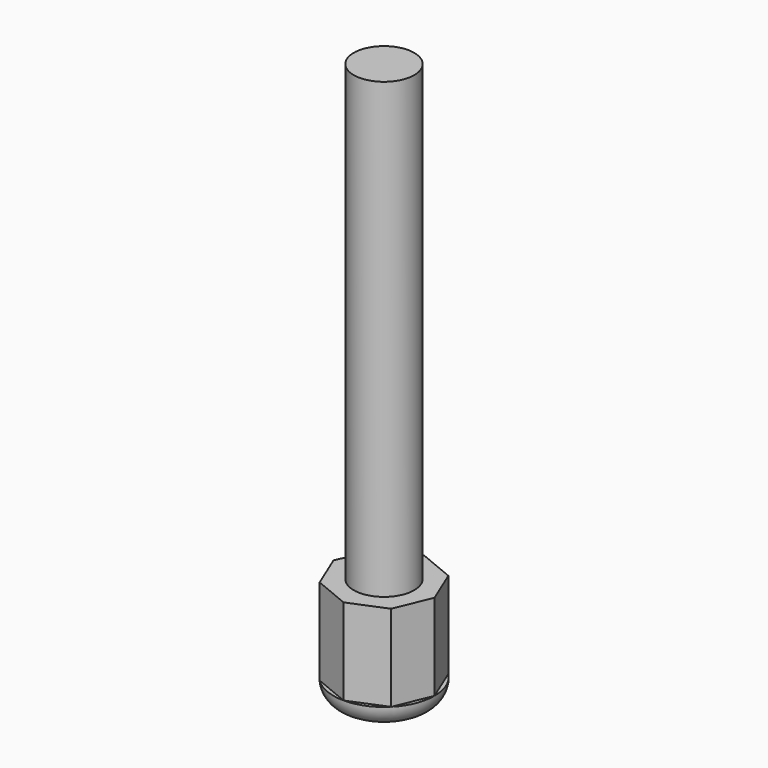
from build123d import *

# Parameters (mm, degrees)
F0_R     = 7
F1_DEPTH = 105
F2_R     = 11.7037675531
F2_R_2   = 7
F3_DEPTH = 25
F4_R     = 5
F6_DEPTH = 20
F7_DEPTH = 3


with BuildPart() as f1:
    # F0 (on Top) → F1 (new body)
    with BuildSketch(Plane.XY):
        with Locations((-4.6541057527, 0)):
            Circle(F0_R)
    extrude(amount=F1_DEPTH)

    # F2 (on face) → F3 (join)
    with BuildSketch(Plane(origin=(0, 0, 0), x_dir=(1, 0, 0), z_dir=(0, 0, -1))):
        with Locations((-4.6541057527, 0)):
            Circle(F2_R)
        with Locations((-4.6541057527, 0)):
            Circle(F2_R_2, mode=Mode.SUBTRACT)
        with Locations((-4.6541057527, 0)):
            Circle(F2_R_2)
    extrude(amount=F3_DEPTH)

    # F4
    f4_edges = [f1.edges().sort_by_distance(p)[0] for p in [
        (-16.357873, 0, -25),
    ]]
    fillet(f4_edges, radius=F4_R)

    # F5 (on face) → F6 (cut)
    with BuildSketch(Plane.XY):
        with BuildLine():
            Line((-12.4576410745, 8.2758134023), (-4.6541057527, 11.7037675531))
            ThreePointArc((-4.6541057527, 11.7037675531), (-9.1329436915, 10.8128712956), (-12.929919155, 8.2758134023))
            Line((-12.929919155, 8.2758134023), (-12.4576410745, 8.2758134023))
        make_face()
        with BuildLine():
            ThreePointArc((-12.929919155, 8.2758134023), (-15.4669770483, 4.4788379388), (-16.3578733058, 0))
            Line((-16.3578733058, 0), (-12.929919155, 7.727174844))
            Line((-12.929919155, 7.727174844), (-12.929919155, 8.2758134023))
        make_face()
        with BuildLine():
            ThreePointArc((3.6217076495, 8.2758134023), (-0.1752678139, 10.8128712956), (-4.6541057527, 11.7037675531))
            Line((-4.6541057527, 11.7037675531), (3.6217076495, 8.2758134023))
        make_face()
        with BuildLine():
            Line((3.6217076495, 8.2758134023), (7.0496618004, 0))
            ThreePointArc((7.0496618004, 0), (6.1587655429, 4.4788379388), (3.6217076495, 8.2758134023))
        make_face()
        with BuildLine():
            ThreePointArc((3.6217076495, -8.2758134023), (6.1587655429, -4.4788379388), (7.0496618004, 0))
            Line((7.0496618004, 0), (3.6217076495, -8.2758134023))
        make_face()
        with BuildLine():
            Line((3.6217076495, -8.2758134023), (-4.6541057527, -11.7037675531))
            ThreePointArc((-4.6541057527, -11.7037675531), (-0.1752678139, -10.8128712956), (3.6217076495, -8.2758134023))
        make_face()
        with BuildLine():
            Line((-12.929919155, -8.2758134023), (-16.3578733058, 0))
            ThreePointArc((-16.3578733058, 0), (-15.4669770483, -4.4788379388), (-12.929919155, -8.2758134023))
        make_face()
        with BuildLine():
            ThreePointArc((-12.929919155, -8.2758134023), (-9.1329436915, -10.8128712956), (-4.6541057527, -11.7037675531))
            Line((-4.6541057527, -11.7037675531), (-12.929919155, -8.2758134023))
        make_face()
    extrude(amount=-F6_DEPTH, mode=Mode.SUBTRACT)

    # F7 (cut): a face of the model
    f7_faces = [f1.faces().sort_by_distance(p)[0] for p in [
        (-4.6541057527, 0, -25),
    ]]
    extrude(f7_faces, amount=-F7_DEPTH, mode=Mode.SUBTRACT)


solid = f1.part
